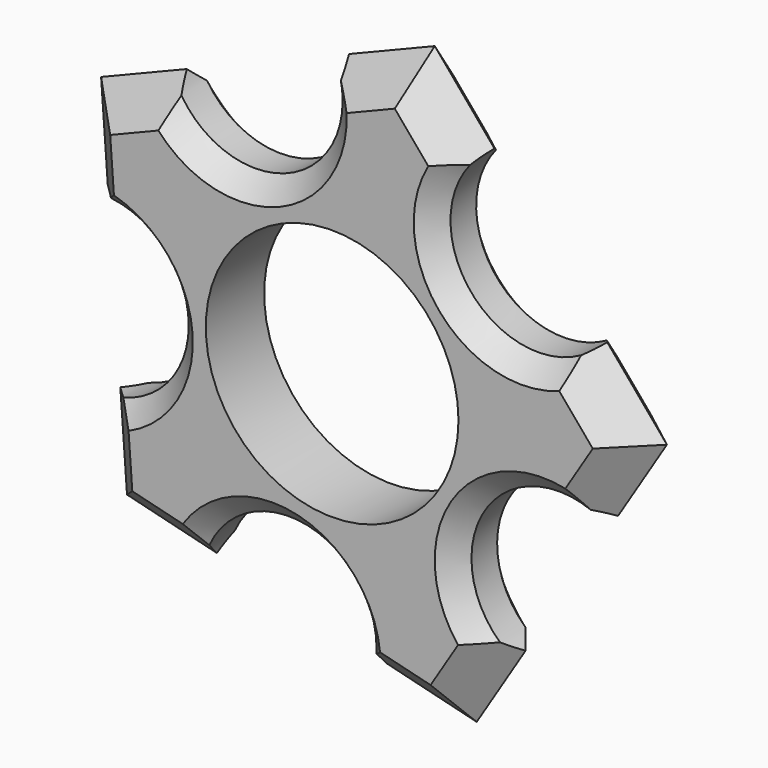
from build123d import *

# Parameters (mm, degrees)
F0_R         = 11
F1_DEPTH     = 6.35
F2_SIZE      = 3.17499
F3_T2_ANGLE  = 199.5715846066
F3_T4_ANGLE  = 199.5715846066
F3_T6_ANGLE  = 199.5715846066
F3_T8_ANGLE  = 199.5715846066
F3_T10_ANGLE = 199.5715846066
F3_T12_ANGLE = 199.5715846066
F3_T14_ANGLE = 199.5715846066
F3_T16_ANGLE = 199.5715846066
F3_T18_ANGLE = 199.5715846066
F3_T20_ANGLE = 199.5715846066


# Not quite as in the source:
# - a fillet or chamfer that OpenCascade refuses, or shapes differently, is made with other operations: its cross-section is extruded or revolved along the edge and cut away or added
# - a fillet or chamfer is up to 0.001 mm smaller than in the source, because OpenCascade refuses the exact size


with BuildPart() as f1:
    # F0 (on Front) → F1 (new body)
    with BuildSketch(Plane.XZ):
        with BuildLine():
            Line((11.5903794876, 19.7357752055), (6.395639386, 25.8985348046))
            Line((6.395639386, 25.8985348046), (-1.0707562618, 22.8624408289))
            ThreePointArc((-1.0707562618, 22.8624408289), (-0.6511189694, 21.4544603732), (-0.5094848211, 19.9921183513))
            ThreePointArc((-0.5094848211, 19.9921183513), (-6.6671427992, 12.5137524996), (-15.1882133804, 17.1217958736))
            Line((-15.1882133804, 17.1217958736), (-22.6546090282, 14.085701898))
            Line((-22.6546090282, 14.085701898), (-22.0743552105, 6.0465330289))
            ThreePointArc((-22.0743552105, 6.0465330289), (-16.3352014079, 4.025037517), (-13.9057833978, -1.5536951891))
            ThreePointArc((-13.9057833978, -1.5536951891), (-15.9470506916, -6.744277179), (-20.977211585, -9.1539234072))
            Line((-20.977211585, -9.1539234072), (-20.3969577673, -17.1930922762))
            Line((-20.3969577673, -17.1930922762), (-12.5719455381, -19.125477903))
            ThreePointArc((-12.5719455381, -19.125477903), (-4.2540087238, -13.3881176755), (2.4458190468, -20.9523547863))
            ThreePointArc((2.4458190468, -20.9523547863), (2.3900561576, -21.8725270157), (2.2235836317, -22.7792316697))
            Line((2.2235836317, -22.7792316697), (10.0485958609, -24.7116172964))
            Line((10.0485958609, -24.7116172964), (14.3044655632, -17.866728424))
            ThreePointArc((14.3044655632, -17.866728424), (11.8568074939, -7.3720740717), (22.3514618462, -4.9244160023))
            Line((22.3514618462, -4.9244160023), (26.6073315486, 1.9204728701))
            Line((26.6073315486, 1.9204728701), (21.412591447, 8.0832324691))
            ThreePointArc((21.412591447, 8.0832324691), (10.6752140991, 8.9983978576), (11.5903794876, 19.7357752055))
        make_face()
        Circle(F0_R, mode=Mode.SUBTRACT)
    extrude(amount=F1_DEPTH)

    # F2 (size 3.175 in the source; OpenCascade refuses exactly that, so slightly less here)
    f2_edges = [f1.edges().sort_by_distance(p)[0] for p in [
        (24.479397, -6.35, -1.501972),
        (24.009961, -6.35, 5.001853),
        (8.993009, -6.35, 22.817155),
        (2.662442, -6.35, 24.380488),
        (-18.921411, -6.35, 15.603749),
        (-22.364482, -6.35, 10.066117),
        (-20.687085, -6.35, -13.173508),
        (-16.484452, -6.35, -18.159285),
        (24.009961, 0, 5.001853),
        (24.479397, 0, -1.501972),
        (8.993009, 0, 22.817155),
        (2.662442, 0, 24.380488),
        (-18.921411, 0, 15.603749),
        (-22.364482, 0, 10.066117),
        (-20.687085, 0, -13.173508),
        (-16.484452, 0, -18.159285),
        (6.13609, 0, -23.745424),
        (12.176531, 0, -21.289173),
        (12.176531, -6.35, -21.289173),
        (6.13609, -6.35, -23.745424),
    ]]
    chamfer(f2_edges, length=F2_SIZE)

    # F3: chamfer of 1.778 on 10 edges, made by hand

    # F3_s1 → F3_t2 (revolve, cut)
    with BuildSketch(Plane(origin=(19.7071717725, 0, -7.9965849701), x_dir=(0, 1, 0), z_dir=(0.9266214967, 0, -0.3759954812))):
        Polygon((-1.778, -11.2881506475), (0, -13.0661506475), (0, -11.2881506475), align=None)
    revolve(axis=Axis((18.3279637047, 0, -11.3955722132), (0, 1, 0)), revolution_arc=F3_T2_ANGLE, mode=Mode.SUBTRACT)

    # F3_s3 → F3_t4 (revolve, cut)
    with BuildSketch(Plane(origin=(19.7071717725, 0, -7.9965849701), x_dir=(0, 1, 0), z_dir=(0.9266214967, 0, -0.3759954812))):
        Polygon((-4.572, -11.2881506475), (-6.35, -13.0661506475), (-6.35, -11.2881506475), align=None)
    revolve(axis=Axis((18.3279637047, -6.35, -11.3955722132), (0, 1, 0)), revolution_arc=F3_T4_ANGLE, mode=Mode.SUBTRACT)

    # F3_s5 → F3_t6 (revolve, cut)
    with BuildSketch(Plane(origin=(-8.534063628, 0, -19.4804452837), x_dir=(0, 1, 0), z_dir=(-0.4012674626, 0, -0.915960929))):
        Polygon((-6.35, 13.0661506475), (-4.572, 11.2881506475), (-6.35, 11.2881506475), align=None)
    revolve(axis=Axis((-5.1741809532, -6.35, -20.9523547863), (0, -1, 0)), revolution_arc=F3_T6_ANGLE, mode=Mode.SUBTRACT)

    # F3_s7 → F3_t8 (revolve, cut)
    with BuildSketch(Plane(origin=(-1.5153532552, 0, -21.2137147847), x_dir=(0, 1, 0), z_dir=(-0.0712511627, 0, -0.9974584061))):
        Polygon((0, -13.0661506475), (-1.778, -11.2881506475), (0, -11.2881506475), align=None)
    revolve(axis=Axis((-5.1741809532, 0, -20.9523547863), (0, 1, 0)), revolution_arc=F3_T8_ANGLE, mode=Mode.SUBTRACT)

    # F3_s9 → F3_t10 (revolve, cut)
    with BuildSketch(Plane(origin=(-21.1641751195, 0, 2.0965881732), x_dir=(0, 1, 0), z_dir=(-0.9951290754, 0, 0.0985805418))):
        Polygon((-6.35, 13.0661506475), (-4.572, 11.2881506475), (-6.35, 11.2881506475), align=None)
    revolve(axis=Axis((-21.5257833978, -6.35, -1.5536951891), (0, -1, 0)), revolution_arc=F3_T10_ANGLE, mode=Mode.SUBTRACT)

    # F3_s11 → F3_t12 (revolve, cut)
    with BuildSketch(Plane(origin=(-20.6437115892, 0, -5.1142117945), x_dir=(0, 1, 0), z_dir=(-0.9706571369, 0, -0.2404677161))):
        Polygon((0, -13.0661506475), (-1.778, -11.2881506475), (0, -11.2881506475), align=None)
    revolve(axis=Axis((-21.5257833978, 0, -1.5536951891), (0, 1, 0)), revolution_arc=F3_T12_ANGLE, mode=Mode.SUBTRACT)

    # F3_s13 → F3_t14 (revolve, cut)
    with BuildSketch(Plane(origin=(-4.5461159397, 0, 20.7762080351), x_dir=(0, 1, 0), z_dir=(-0.2137561292, 0, 0.9768870545))):
        Polygon((-6.35, 13.0661506475), (-4.572, 11.2881506475), (-6.35, 11.2881506475), align=None)
    revolve(axis=Axis((-8.1294848211, -6.35, 19.9921183513), (0, -1, 0)), revolution_arc=F3_T14_ANGLE, mode=Mode.SUBTRACT)

    # F3_s15 → F3_t16 (revolve, cut)
    with BuildSketch(Plane(origin=(-11.2431621609, 0, 18.0529580701), x_dir=(0, 1, 0), z_dir=(-0.5286479394, 0, 0.8488411843))):
        Polygon((0, -13.0661506475), (-1.778, -11.2881506475), (0, -11.2881506475), align=None)
    revolve(axis=Axis((-8.1294848211, 0, 19.9921183513), (0, 1, 0)), revolution_arc=F3_T16_ANGLE, mode=Mode.SUBTRACT)

    # F3_s17 → F3_t18 (revolve, cut)
    with BuildSketch(Plane(origin=(13.6950552327, 0, 16.2715534792), x_dir=(0, 1, 0), z_dir=(0.6439347423, 0, 0.7650804191))):
        Polygon((-6.35, -13.0661506475), (-4.572, -11.2881506475), (-6.35, -11.2881506475), align=None)
    revolve(axis=Axis((16.5014854673, -6.35, 13.9095038373), (0, 1, 0)), revolution_arc=F3_T18_ANGLE, mode=Mode.SUBTRACT)

    # F3_s19 → F3_t20 (revolve, cut)
    with BuildSketch(Plane(origin=(13.6950552327, 0, 16.2715534792), x_dir=(0, 1, 0), z_dir=(0.6439347423, 0, 0.7650804191))):
        Polygon((0, -13.0661506475), (-1.778, -11.2881506475), (0, -11.2881506475), align=None)
    revolve(axis=Axis((16.5014854673, 0, 13.9095038373), (0, 1, 0)), revolution_arc=F3_T20_ANGLE, mode=Mode.SUBTRACT)


solid = f1.part
